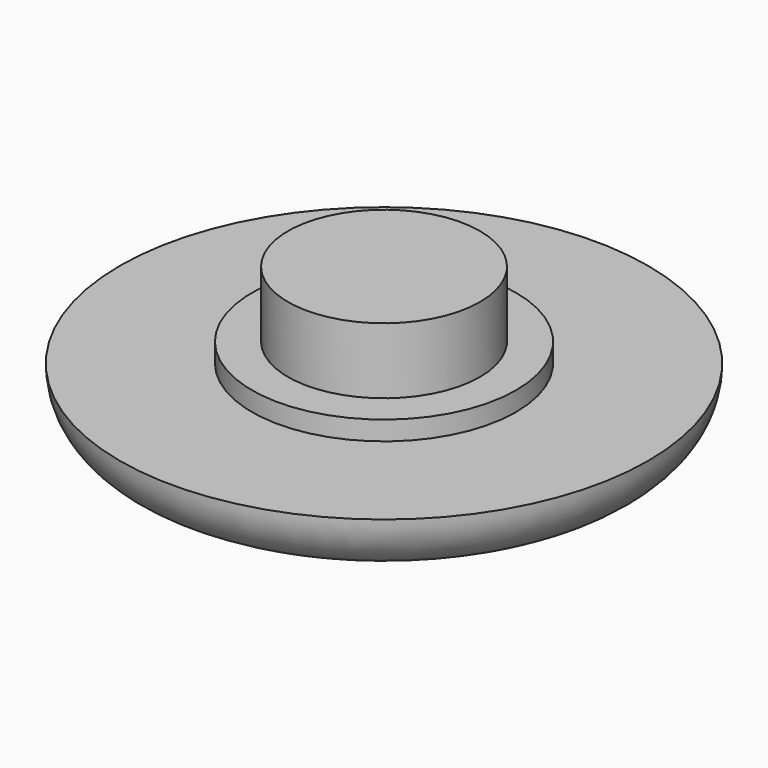
from build123d import *

# Parameters (mm, degrees)
F0_R      = 11
F0_R_2    = 5.5
F1_DEPTH  = 2.5
F0_R_3    = 4
F2_DEPTH  = 3.3
F3_DEPTH  = 6.05
F4_R      = 2.49999
F7_W      = 0.9174569654
F7_H      = 1.9074306578
F8_DEPTH  = 1
F9_W      = 10.9082679264
F9_H      = 0.01
F9_W_2    = 0.01
F9_H_2    = 1.80521388
F9_W_3    = 2.0817320736
F9_H_3    = 3.4049642272
F10_DEPTH = 0.1


# Not quite as in the source:
# - a fillet or chamfer is up to 0.001 mm smaller than in the source, because OpenCascade refuses the exact size


with BuildPart() as f1:
    # F0 (on Top) → F1 (new body)
    with BuildSketch(Plane.XY):
        Circle(F0_R)
        Circle(F0_R_2, mode=Mode.SUBTRACT)
    extrude(amount=F1_DEPTH)

    # F0 (on Top) → F2 (join, through all)
    with BuildSketch(Plane.XY):
        Circle(F0_R_2)
        Circle(F0_R_3, mode=Mode.SUBTRACT)
    extrude(amount=F2_DEPTH)

    # F0 (on Top) → F3 (join, through all)
    with BuildSketch(Plane.XY):
        Circle(F0_R_3)
    extrude(amount=F3_DEPTH)

    # F4 (radius 2.5 in the source; OpenCascade refuses exactly that, so slightly less here)
    f4_edges = [f1.edges().sort_by_distance(p)[0] for p in [
        (-11, 0, 0),
    ]]
    fillet(f4_edges, radius=F4_R)

    # F7 (on face) → F8 (cut)
    with BuildSketch(Plane(origin=(0, 0, 0), x_dir=(1, 0, 0), z_dir=(0, 0, -1))):
        with Locations((-5.6969438194, 0.9537153289)):
            Rectangle(F7_W, F7_H)
        with BuildLine():
            Line((-5.2382153367, 0), (-6.1556723021, 0))
            Line((-6.1556723021, 0), (-6.1556723021, -2.1458544496))
            add(Edge.make_bspline(
                [(-6.285858404, -2.7333488222), (-6.1556723021, -2.5454074314), (-6.1556723021, -2.1458544496)],
                knots=[0, 0, 0, 1, 1, 1], degree=2))
            add(Edge.make_bspline(
                [(-6.7180762624, -2.9212902129), (-6.4160445059, -2.9212902129), (-6.285858404, -2.7333488222)],
                knots=[0, 0, 0, 1, 1, 1], degree=2))
            add(Edge.make_bspline(
                [(-7.1498207167, -2.8625881161), (-6.9131187132, -2.9212902129), (-6.7180762624, -2.9212902129)],
                knots=[0, 0, 0, 1, 1, 1], degree=2))
            Line((-7.1498207167, -2.8625881161), (-7.1498207167, -3.6257153753))
            add(Edge.make_bspline(
                [(-6.6082465328, -3.6910451282), (-6.9187995613, -3.6910451282), (-7.1498207167, -3.6257153753)],
                knots=[0, 0, 0, 1, 1, 1], degree=2))
            add(Edge.make_bspline(
                [(-5.5842736658, -3.2943325704), (-5.9303319948, -3.6910451282), (-6.6082465328, -3.6910451282)],
                knots=[0, 0, 0, 1, 1, 1], degree=2))
            add(Edge.make_bspline(
                [(-5.2382153367, -2.1401736015), (-5.2382153367, -2.8976200126), (-5.5842736658, -3.2943325704)],
                knots=[0, 0, 0, 1, 1, 1], degree=2))
            Line((-5.2382153367, -2.1401736015), (-5.2382153367, 0))
        make_face()
        with BuildLine():
            Line((4.6739177604, 1.9074306578), (4.6739177604, 0))
            Line((4.6739177604, 0), (7.4127629667, 0))
            add(Edge.make_bspline(
                [(7.5900864431, 0.1761922044), (7.5124036184, 0.0699852174), (7.4127629667, 0)],
                knots=[0, 0, 0, 0.4273284972, 0.4273284972, 0.4273284972], degree=2))
            add(Edge.make_bspline(
                [(7.7718735818, 0.8129205937), (7.7718735818, 0.4247293081), (7.5900864431, 0.1761922044)],
                knots=[0, 0, 0, 1, 1, 1], degree=2))
            add(Edge.make_bspline(
                [(7.3562248637, 1.6456382419), (7.7718735818, 1.3838458261), (7.7718735818, 0.8129205937)],
                knots=[0, 0, 0, 1, 1, 1], degree=2))
            add(Edge.make_bspline(
                [(6.0202787562, 1.9074306578), (6.9405761456, 1.9074306578), (7.3562248637, 1.6456382419)],
                knots=[0, 0, 0, 1, 1, 1], degree=2))
            Line((6.0202787562, 1.9074306578), (4.6739177604, 1.9074306578))
        make_face()
        with BuildLine():
            Line((6.1234808297, 0.1937081527), (5.5913747259, 0.1937081527))
            Line((5.5913747259, 0.1937081527), (5.5913747259, 1.1556650948))
            Line((5.5913747259, 1.1556650948), (6.0733000049, 1.1556650948))
            add(Edge.make_bspline(
                [(6.6489592774, 1.0477289812), (6.4671721387, 1.1556650948), (6.0733000049, 1.1556650948)],
                knots=[0, 0, 0, 1, 1, 1], degree=2))
            add(Edge.make_bspline(
                [(6.830746416, 0.69078236), (6.830746416, 0.9397928676), (6.6489592774, 1.0477289812)],
                knots=[0, 0, 0, 1, 1, 1], degree=2))
            add(Edge.make_bspline(
                [(6.6636348016, 0.3092187304), (6.830746416, 0.4247293081), (6.830746416, 0.69078236)],
                knots=[0, 0, 0, 1, 1, 1], degree=2))
            add(Edge.make_bspline(
                [(6.1234808297, 0.1937081527), (6.4965231871, 0.1937081527), (6.6636348016, 0.3092187304)],
                knots=[0, 0, 0, 1, 1, 1], degree=2))
        make_face(mode=Mode.SUBTRACT)
        with BuildLine():
            Line((7.4127629667, 0), (4.6739177604, 0))
            Line((4.6739177604, 0), (4.6739177604, -2.4185351576))
            Line((4.6739177604, -2.4185351576), (6.2920126561, -2.4185351576))
            add(Edge.make_bspline(
                [(7.4537460891, -2.0871523527), (7.0257888669, -2.4185351576), (6.2920126561, -2.4185351576)],
                knots=[0, 0, 0, 1, 1, 1], degree=2))
            add(Edge.make_bspline(
                [(7.8817033114, -1.1640145392), (7.8817033114, -1.7557695479), (7.4537460891, -2.0871523527)],
                knots=[0, 0, 0, 1, 1, 1], degree=2))
            add(Edge.make_bspline(
                [(7.6994427687, -0.4950946774), (7.8817033114, -0.7464722051), (7.8817033114, -1.1640145392)],
                knots=[0, 0, 0, 1, 1, 1], degree=2))
            add(Edge.make_bspline(
                [(7.1062675481, -0.1518767724), (7.5171822261, -0.2437171497), (7.6994427687, -0.4950946774)],
                knots=[0, 0, 0, 1, 1, 1], degree=2))
            Line((7.1062675481, -0.1518767724), (7.1062675481, -0.122525724))
            add(Edge.make_bspline(
                [(7.4127629667, 0), (7.2792325279, -0.0937885956), (7.1062675481, -0.122525724)],
                knots=[0.4273284972, 0.4273284972, 0.4273284972, 1, 1, 1], degree=2))
        make_face()
        with BuildLine():
            Line((5.5913747259, -1.6610887465), (5.5913747259, -0.533440402))
            Line((5.5913747259, -0.533440402), (6.1594595342, -0.533440402))
            add(Edge.make_bspline(
                [(6.9282676415, -1.0721741619), (6.9282676415, -0.533440402), (6.1594595342, -0.533440402)],
                knots=[0, 0, 0, 1, 1, 1], degree=2))
            add(Edge.make_bspline(
                [(6.7479007148, -1.5162271204), (6.9282676415, -1.3713654942), (6.9282676415, -1.0721741619)],
                knots=[0, 0, 0, 1, 1, 1], degree=2))
            add(Edge.make_bspline(
                [(6.1888105826, -1.6610887465), (6.5675337882, -1.6610887465), (6.7479007148, -1.5162271204)],
                knots=[0, 0, 0, 1, 1, 1], degree=2))
            Line((6.1888105826, -1.6610887465), (5.5913747259, -1.6610887465))
        make_face(mode=Mode.SUBTRACT)
        with BuildLine():
            add(Edge.make_bspline(
                [(-0.3341412716, 0), (-0.2793910242, 0.9026419622), (0.1926754308, 1.4060958144)],
                knots=[0.1159799575, 0.1159799575, 0.1159799575, 1, 1, 1], degree=2))
            Line((-0.3341412716, 0), (0.629649983, 0))
            add(Edge.make_bspline(
                [(0.8985208052, 0.8432184502), (0.6706907109, 0.5412562469), (0.629649983, 0)],
                knots=[0, 0, 0, 0.8198625691, 0.8198625691, 0.8198625691], degree=2))
            add(Edge.make_bspline(
                [(1.7236639892, 1.2115267676), (1.1764089572, 1.2115267676), (0.8985208052, 0.8432184502)],
                knots=[0, 0, 0, 1, 1, 1], degree=2))
            add(Edge.make_bspline(
                [(2.8066188149, 0), (2.7177954406, 1.2115267676), (1.7236639892, 1.2115267676)],
                knots=[0.0893477157, 0.0893477157, 0.0893477157, 1, 1, 1], degree=2))
            Line((2.8066188149, 0), (3.7697905547, 0))
            add(Edge.make_bspline(
                [(3.2489716996, 1.4013617744), (3.7143429717, 0.8955415655), (3.7697905547, 0)],
                knots=[0, 0, 0, 0.880853017, 0.880853017, 0.880853017], degree=2))
            add(Edge.make_bspline(
                [(1.7236639892, 1.9756008348), (2.7206528278, 1.9756008348), (3.2489716996, 1.4013617744)],
                knots=[0, 0, 0, 1, 1, 1], degree=2))
            add(Edge.make_bspline(
                [(0.1926754308, 1.4060958144), (0.7266751506, 1.9756008348), (1.7236639892, 1.9756008348)],
                knots=[0, 0, 0, 1, 1, 1], degree=2))
        make_face()
        with BuildLine():
            Line((0.629649983, 0), (-0.3341412716, 0))
            add(Edge.make_bspline(
                [(-0.341324289, -0.2437171497), (-0.341324289, -0.1184230803), (-0.3341412716, 0)],
                knots=[0, 0, 0, 0.1159799575, 0.1159799575, 0.1159799575], degree=2))
            add(Edge.make_bspline(
                [(0.1912552188, -1.901104578), (-0.341324289, -1.3240250936), (-0.341324289, -0.2437171497)],
                knots=[0, 0, 0, 1, 1, 1], degree=2))
            add(Edge.make_bspline(
                [(1.7179831412, -2.4781840625), (0.7238347266, -2.4781840625), (0.1912552188, -1.901104578)],
                knots=[0, 0, 0, 1, 1, 1], degree=2))
            add(Edge.make_bspline(
                [(3.2447110635, -1.901104578), (2.7121315557, -2.4781840625), (1.7179831412, -2.4781840625)],
                knots=[0, 0, 0, 1, 1, 1], degree=2))
            add(Edge.make_bspline(
                [(3.7772905713, -0.2493979978), (3.7772905713, -1.3240250936), (3.2447110635, -1.901104578)],
                knots=[0, 0, 0, 1, 1, 1], degree=2))
            add(Edge.make_bspline(
                [(3.7697905547, 0), (3.7772905713, -0.1211338029), (3.7772905713, -0.2493979978)],
                knots=[0.880853017, 0.880853017, 0.880853017, 1, 1, 1], degree=2))
            Line((3.7697905547, 0), (2.8066188149, 0))
            add(Edge.make_bspline(
                [(2.8153336292, -0.2493979978), (2.8153336292, -0.1188677073), (2.8066188149, 0)],
                knots=[0, 0, 0, 0.0893477157, 0.0893477157, 0.0893477157], degree=2))
            add(Edge.make_bspline(
                [(1.7179831412, -1.7084291472), (2.8153336292, -1.7084291472), (2.8153336292, -0.2493979978)],
                knots=[0, 0, 0, 1, 1, 1], degree=2))
            add(Edge.make_bspline(
                [(0.8956803811, -1.3415410418), (1.1707281091, -1.7084291472), (1.7179831412, -1.7084291472)],
                knots=[0, 0, 0, 1, 1, 1], degree=2))
            add(Edge.make_bspline(
                [(0.6206326531, -0.2493979978), (0.6206326531, -0.9746529364), (0.8956803811, -1.3415410418)],
                knots=[0, 0, 0, 1, 1, 1], degree=2))
            add(Edge.make_bspline(
                [(0.629649983, 0), (0.6206326531, -0.118922992), (0.6206326531, -0.2493979978)],
                knots=[0.8198625691, 0.8198625691, 0.8198625691, 1, 1, 1], degree=2))
        make_face()
        with BuildLine():
            Line((-4.1493861208, 1.9074306578), (-4.1493861208, 0))
            Line((-4.1493861208, 0), (-3.2319291553, 0))
            Line((-3.2319291553, 0), (-3.2319291553, 1.1556650948))
            Line((-3.2319291553, 1.1556650948), (-2.9535675992, 1.1556650948))
            add(Edge.make_bspline(
                [(-2.2988498577, 1.0254789929), (-2.5104614488, 1.1556650948), (-2.9535675992, 1.1556650948)],
                knots=[0, 0, 0, 1, 1, 1], degree=2))
            add(Edge.make_bspline(
                [(-2.0872382666, 0.5875802864), (-2.0872382666, 0.8952928909), (-2.2988498577, 1.0254789929)],
                knots=[0, 0, 0, 1, 1, 1], degree=2))
            add(Edge.make_bspline(
                [(-2.2941158176, 0.1321656318), (-2.0872382666, 0.2770272579), (-2.0872382666, 0.5875802864)],
                knots=[0, 0, 0, 1, 1, 1], degree=2))
            add(Edge.make_bspline(
                [(-2.698691477, 0), (-2.4397484519, 0.0301894622), (-2.2941158176, 0.1321656318)],
                knots=[0.2960442854, 0.2960442854, 0.2960442854, 1, 1, 1], degree=2))
            Line((-2.698691477, 0), (-1.3266566892, 0))
            add(Edge.make_bspline(
                [(-1.161260029, 0.6112504868), (-1.161260029, 0.272396569), (-1.3266566892, 0)],
                knots=[0, 0, 0, 0.8880666067, 0.8880666067, 0.8880666067], degree=2))
            add(Edge.make_bspline(
                [(-1.5840098072, 1.5864627411), (-1.161260029, 1.2654948244), (-1.161260029, 0.6112504868)],
                knots=[0, 0, 0, 1, 1, 1], degree=2))
            add(Edge.make_bspline(
                [(-2.8891846543, 1.9074306578), (-2.0067595854, 1.9074306578), (-1.5840098072, 1.5864627411)],
                knots=[0, 0, 0, 1, 1, 1], degree=2))
            Line((-2.8891846543, 1.9074306578), (-4.1493861208, 1.9074306578))
        make_face()
        with BuildLine():
            Line((-3.2319291553, 0), (-4.1493861208, 0))
            Line((-4.1493861208, 0), (-4.1493861208, -2.4185351576))
            Line((-4.1493861208, -2.4185351576), (-3.2319291553, -2.4185351576))
            Line((-3.2319291553, -2.4185351576), (-3.2319291553, -0.7587807093))
            Line((-3.2319291553, -0.7587807093), (-2.7443230282, -0.7587807093))
            Line((-2.7443230282, -0.7587807093), (-1.7113554851, -2.4185351576))
            Line((-1.7113554851, -2.4185351576), (-0.6935368702, -2.4185351576))
            add(Edge.make_bspline(
                [(-1.9660468408, -0.533440402), (-0.9889409705, -1.9924715513), (-0.6935368702, -2.4185351576)],
                knots=[0, 0, 0, 1, 1, 1], degree=2))
            add(Edge.make_bspline(
                [(-1.3709780041, -0.0676108592), (-1.5806959791, -0.3649085755), (-1.9660468408, -0.533440402)],
                knots=[0, 0, 0, 1, 1, 1], degree=2))
            add(Edge.make_bspline(
                [(-1.3266566892, 0), (-1.3475035595, -0.034333317), (-1.3709780041, -0.0676108592)],
                knots=[0.8880666067, 0.8880666067, 0.8880666067, 1, 1, 1], degree=2))
            Line((-1.3266566892, 0), (-2.698691477, 0))
            add(Edge.make_bspline(
                [(-2.936525055, -0.0126959944), (-2.8075883881, -0.0126959944), (-2.698691477, 0)],
                knots=[0, 0, 0, 0.2960442854, 0.2960442854, 0.2960442854], degree=2))
            Line((-2.936525055, -0.0126959944), (-3.2319291553, -0.0126959944))
            Line((-3.2319291553, -0.0126959944), (-3.2319291553, 0))
        make_face()
    extrude(amount=-F8_DEPTH, mode=Mode.SUBTRACT)

    # F9 (on face) → F10 (join)
    with BuildSketch(Plane(origin=(0, 0, 0), x_dir=(1, 0, 0), z_dir=(0, 0, -1))):
        with Locations((0.5191841628, 0.5439160942)):
            Rectangle(F9_W, F9_H)
        with Locations((5.9783181261, 1.4515230342)):
            Rectangle(F9_W_2, F9_H_2)
        with Locations((5.9783181261, 0.5439160942)):
            Rectangle(F9_W_2, F9_H)
        with Locations((7.0241841628, 0.5439160942)):
            Rectangle(F9_W_3, F9_H)
        with Locations((5.9783181261, -1.1635660194)):
            Rectangle(F9_W_2, F9_H_3)
    extrude(amount=-F10_DEPTH)


solid = f1.part
